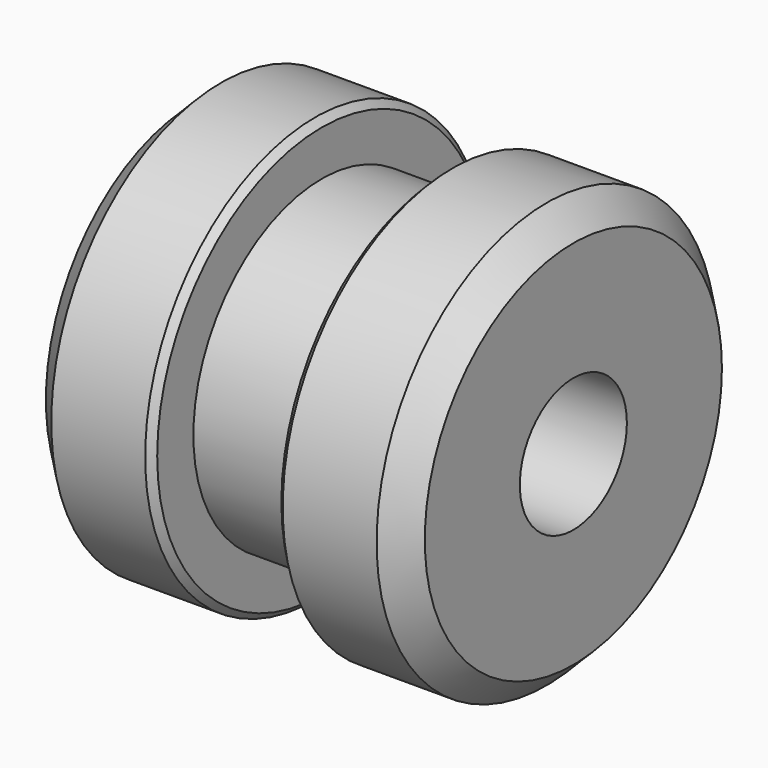
from build123d import *

# Parameters (mm, degrees)
F2_SIZE = 1


# Not quite as in the source:
# - a fillet or chamfer that OpenCascade refuses, or shapes differently, is made with other operations: its cross-section is extruded or revolved along the edge and cut away or added


with BuildPart() as f1:
    # F0 (on Top) → F1 (revolve)
    with BuildSketch(Plane.XY):
        Polygon((0, 7.94), (0, 1), (8.16, 1), (8.16, 2.5), (14.16, 2.5), (14.16, 7.94), (9.4, 7.94), (9.4, 6), (4.76, 6), (4.76, 7.94), align=None)
    revolve(axis=Axis((7.08, 0, 0), (1, 0, 0)))

    # F2
    f2_edges = [f1.edges().sort_by_distance(p)[0] for p in [
        (0, -7.94, 0),
        (14.16, -7.94, 0),
        (0, -1, 0),
    ]]
    chamfer(f2_edges, length=F2_SIZE)

    # F3: chamfer of 0.25 on 3 edges, made by hand

    # F3_s1 → F3_t2 (revolve, cut)
    with BuildSketch(Plane.XY):
        Polygon((4.51, 7.94), (4.76, 7.69), (4.76, 7.94), align=None)
    revolve(axis=Axis((4.76, 0, 0), (1, 0, 0)), mode=Mode.SUBTRACT)

    # F3_s3 → F3_t4 (revolve, cut)
    with BuildSketch(Plane.XY):
        Polygon((9.4, 7.69), (9.65, 7.94), (9.4, 7.94), align=None)
    revolve(axis=Axis((9.4, 0, 0), (1, 0, 0)), mode=Mode.SUBTRACT)

    # F3_s5 → F3_t6 (revolve, cut)
    with BuildSketch(Plane.XY):
        Polygon((0, 2.1035533906), (0.0732233047, 1.9267766953), (0, 2), align=None)
    revolve(axis=Axis((0, 0, 0), (1, 0, 0)), mode=Mode.SUBTRACT)


solid = f1.part
